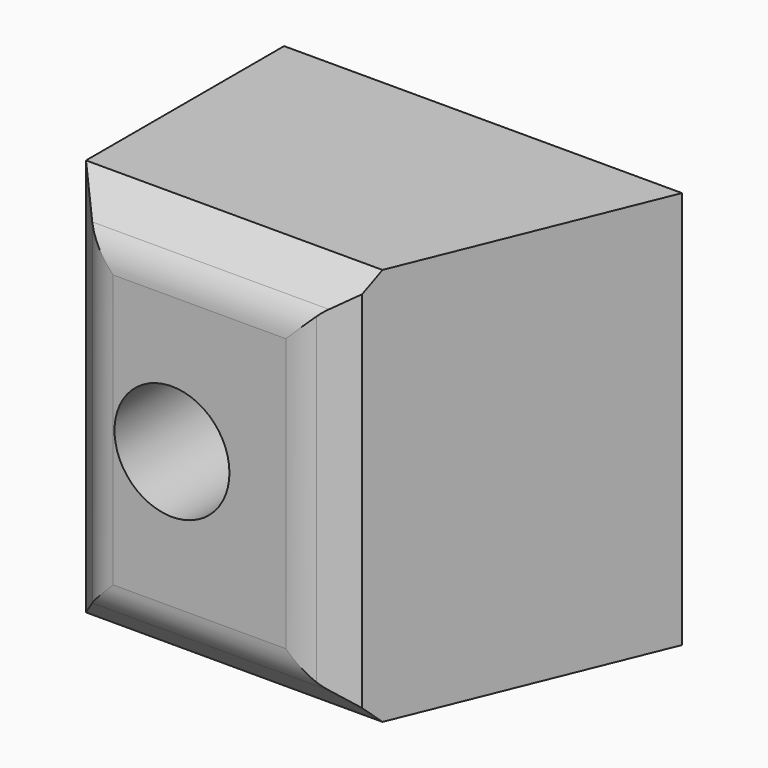
from build123d import *

# Parameters (mm, degrees)
F0_W        = 45
F0_H        = 45
F1_DEPTH    = 33
F3_DEPTH    = 55.8
F4_R        = 6.5
F5_DEPTH    = 68.3
F6_T1_DEPTH = 57.1976554231
F6_T3_DEPTH = 62.61396425
F6_T5_DEPTH = 70.7168298797
F7_R        = 5


# Not quite as in the source:
# - a fillet or chamfer that OpenCascade refuses, or shapes differently, is made with other operations: its cross-section is extruded or revolved along the edge and cut away or added


with BuildPart() as f1:
    # F0 (on Front) → F1 (new body)
    with BuildSketch(Plane.XZ):
        Rectangle(F0_W, F0_H)
    extrude(amount=F1_DEPTH)

    # F2 (on face) → F3 (cut)
    with BuildSketch(Plane.XY.offset(22.5)):
        Polygon((22.5, -33), (22.5, 0), (8.9808255434, -33), align=None)
    extrude(amount=-F3_DEPTH, mode=Mode.SUBTRACT)

    # F4 (on face) → F5 (cut)
    with BuildSketch(Plane.XZ.offset(33)):
        with Locations((-8.7795946747, 0)):
            Circle(F4_R)
    extrude(amount=-F5_DEPTH, mode=Mode.SUBTRACT)

    # F6: chamfer of 5 on 4 edges, made by hand

    # F6_s2 → F6_t1 (cut)
    with BuildSketch(Plane.YZ.offset(-35.3584149398)):
        Polygon((-28, 22.5), (-33, 17.5), (-33, 22.5), align=None)
        Polygon((-28, -22.5), (-33, -17.5), (-33, -22.5), align=None)
    extrude(amount=F6_T1_DEPTH, mode=Mode.SUBTRACT)

    # F6_s4 → F6_t3 (cut)
    with BuildSketch(Plane.XY.offset(-31.306982125)):
        Polygon((10.252665661, -29.8954669522), (5.6258735721, -33), (8.9808255434, -33), align=None)
    extrude(amount=F6_T3_DEPTH, mode=Mode.SUBTRACT)

    # F6_s6 → F6_t5 (cut)
    with BuildSketch(Plane.XY.offset(-35.3584149398)):
        Polygon((-22.5, -28), (-17.5, -33), (-22.5, -33), align=None)
    extrude(amount=F6_T5_DEPTH, mode=Mode.SUBTRACT)

    # F7
    f7_edges = [f1.edges().sort_by_distance(p)[0] for p in [
        (-5.937063, -33, 17.5),
        (5.625874, -33, 0),
        (-5.937063, -33, -17.5),
        (-17.5, -33, 0),
    ]]
    fillet(f7_edges, radius=F7_R)


solid = f1.part
